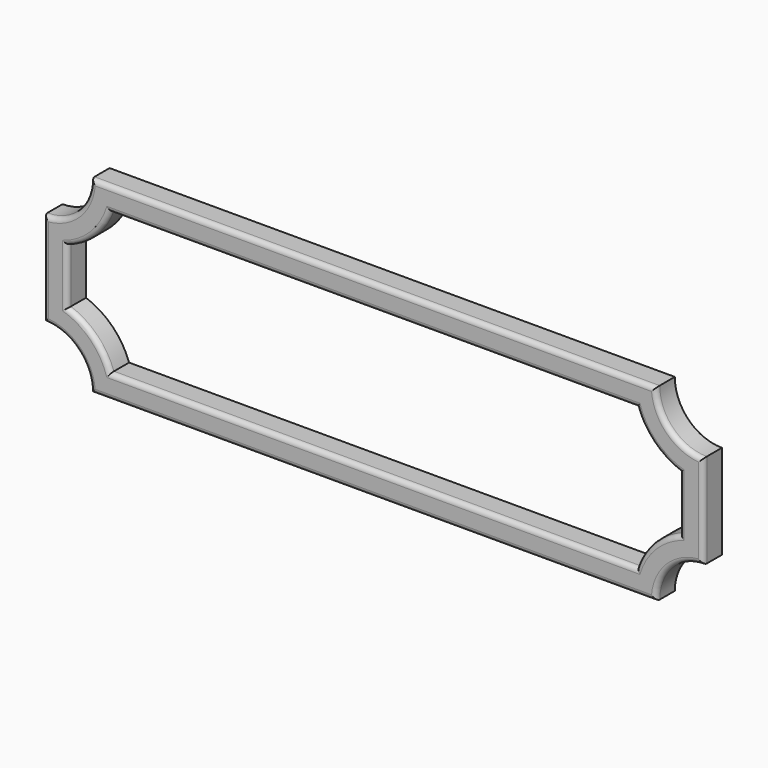
from build123d import *

# Parameters (mm, degrees)
F1_DEPTH = 6.35
F2_R     = 1.27


with BuildPart() as f1:
    # F0 (on Front) → F1 (new body)
    with BuildSketch(Plane.XZ):
        with BuildLine():
            ThreePointArc((-69.85, 25.4), (-70.1243474386, 22.1786073053), (-70.9394877579, 19.05))
            Line((-70.9394877579, 19.05), (70.9394877579, 19.05))
            ThreePointArc((70.9394877579, 19.05), (70.1243474386, 22.1786073053), (69.85, 25.4))
            Line((69.85, 25.4), (-69.85, 25.4))
        make_face()
        with BuildLine():
            Line((-88.9, 12.7), (-88.9, 6.35))
            ThreePointArc((-88.9, 6.35), (-85.6786055668, 6.6243477369), (-82.5499966741, 7.4394889338))
            ThreePointArc((-82.5499966741, 7.4394889338), (-75.4296145712, 11.9296170656), (-70.9394877579, 19.05))
            ThreePointArc((-70.9394877579, 19.05), (-70.1243474386, 22.1786073053), (-69.85, 25.4))
            Line((-69.85, 25.4), (-76.2, 25.4))
            ThreePointArc((-76.2, 25.4), (-79.9197438789, 16.4197438789), (-88.9, 12.7))
        make_face()
        with BuildLine():
            ThreePointArc((-88.9, -12.7), (-79.9197438789, -16.4197438789), (-76.2, -25.4))
            Line((-76.2, -25.4), (-69.85, -25.4))
            ThreePointArc((-69.85, -25.4), (-70.1243475845, -22.1786064547), (-70.9394883332, -19.0499983728))
            ThreePointArc((-70.9394883332, -19.0499983728), (-75.4296151814, -11.9296164554), (-82.5499966741, -7.4394889338))
            ThreePointArc((-82.5499966741, -7.4394889338), (-85.6786055668, -6.6243477369), (-88.9, -6.35))
            Line((-88.9, -6.35), (-88.9, -12.7))
        make_face()
        with BuildLine():
            Line((-88.9, 6.35), (-88.9, -6.35))
            ThreePointArc((-88.9, -6.35), (-85.6786055668, -6.6243477369), (-82.5499966741, -7.4394889338))
            Line((-82.5499966741, -7.4394889338), (-82.5499966741, 7.4394889338))
            ThreePointArc((-82.5499966741, 7.4394889338), (-85.6786055668, 6.6243477369), (-88.9, 6.35))
        make_face()
        with BuildLine():
            ThreePointArc((-70.9394883332, -19.0499983728), (-70.1243475845, -22.1786064547), (-69.85, -25.4))
            Line((-69.85, -25.4), (69.85, -25.4))
            ThreePointArc((69.85, -25.4), (70.1243475845, -22.1786064547), (70.9394883332, -19.0499983728))
            Line((70.9394883332, -19.0499983728), (-70.9394883332, -19.0499983728))
        make_face()
        with BuildLine():
            ThreePointArc((70.9394883332, -19.0499983728), (70.1243475845, -22.1786064547), (69.85, -25.4))
            Line((69.85, -25.4), (76.2, -25.4))
            ThreePointArc((76.2, -25.4), (79.9197438789, -16.4197438789), (88.9, -12.7))
            Line((88.9, -12.7), (88.9, -6.35))
            ThreePointArc((88.9, -6.35), (85.6786073053, -6.6243474386), (82.55, -7.4394877579))
            ThreePointArc((82.55, -7.4394877579), (75.4296164286, -11.9296152082), (70.9394883332, -19.0499983728))
        make_face()
        with BuildLine():
            Line((82.55, 7.4394877579), (82.55, -7.4394877579))
            ThreePointArc((82.55, -7.4394877579), (85.6786073053, -6.6243474386), (88.9, -6.35))
            Line((88.9, -6.35), (88.9, 6.35))
            ThreePointArc((88.9, 6.35), (85.6786073053, 6.6243474386), (82.55, 7.4394877579))
        make_face()
        with BuildLine():
            ThreePointArc((70.9394877579, 19.05), (75.4296158184, 11.9296158184), (82.55, 7.4394877579))
            ThreePointArc((82.55, 7.4394877579), (85.6786073053, 6.6243474386), (88.9, 6.35))
            Line((88.9, 6.35), (88.9, 12.7))
            ThreePointArc((88.9, 12.7), (79.9197438789, 16.4197438789), (76.2, 25.4))
            Line((76.2, 25.4), (69.85, 25.4))
            ThreePointArc((69.85, 25.4), (70.1243474386, 22.1786073053), (70.9394877579, 19.05))
        make_face()
    extrude(amount=F1_DEPTH)

    # F2
    f2_edges = [f1.edges().sort_by_distance(p)[0] for p in [
        (-79.919744, -6.35, 16.419744),
        (-88.9, -6.35, 0),
        (-79.919744, -6.35, -16.419744),
        (0, -6.35, -25.4),
        (0, -6.35, 25.4),
        (79.919744, -6.35, 16.419744),
        (88.9, -6.35, 0),
        (79.919744, -6.35, -16.419744),
        (82.55, -6.35, 0),
        (75.429616, -6.35, 11.929616),
        (0, -6.35, 19.05),
        (-75.429615, -6.35, 11.929617),
        (-82.549997, -6.35, 0),
        (-75.429615, -6.35, -11.929616),
        (0, -6.35, -19.049998),
        (75.429616, -6.35, -11.929615),
    ]]
    fillet(f2_edges, radius=F2_R)


solid = f1.part
